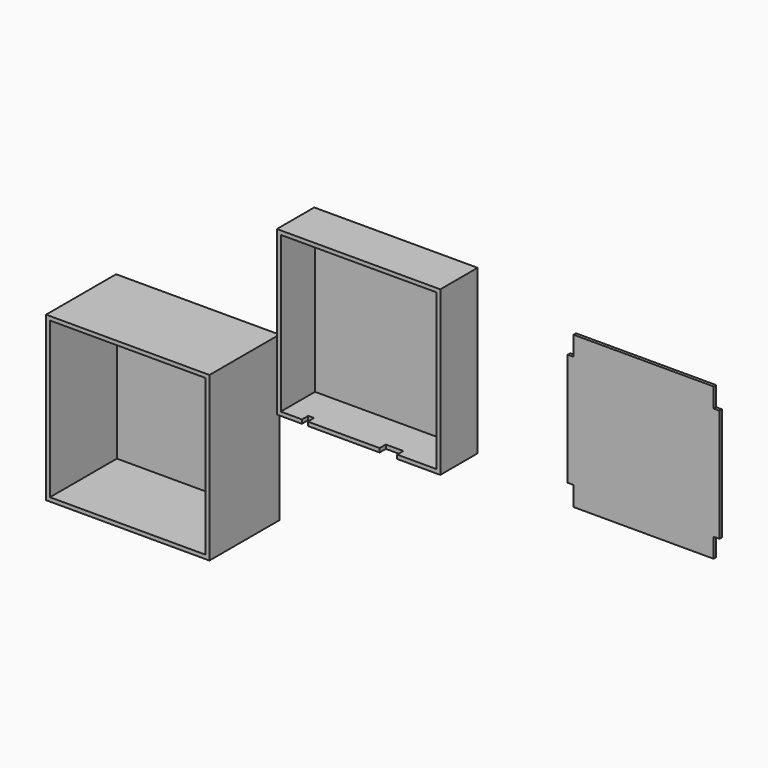
from build123d import *

# Parameters (mm, degrees)
F0_W          = 84
F0_H          = 84
F1_DEPTH      = 24
F2_W          = 80
F2_H          = 80
F3_DEPTH      = 22
F4_W          = 3
F4_H          = 4
F4_W_2        = 9
F5_DEPTH      = 2.5
F7_DEPTH      = 1.6
F8_W          = 84
F8_H          = 84
F8_W_2        = 80
F8_H_2        = 80
F9_DEPTH      = 2
F10_DEPTH     = 45
F11_TEXT_SIZE = 6.5938594684
F12_DEPTH     = 0.5


# Not quite as in the source:
# - Text() gives the source's letters only with a copy of the font that has no kerning and outlines rounded to 1/6400 em; it was checked with that copy


with BuildPart() as f1:
    # F0 (on Front) → F1 (new body)
    with BuildSketch(Plane.XZ):
        Rectangle(F0_W, F0_H)
    extrude(amount=F1_DEPTH)

    # F2 (on face) → F3 (cut)
    with BuildSketch(Plane.XZ.offset(24)):
        Rectangle(F2_W, F2_H)
    extrude(amount=-F3_DEPTH, mode=Mode.SUBTRACT)

    # F4 (on face) → F5 (cut)
    with BuildSketch(Plane(origin=(0, 0, -42), x_dir=(1, 0, 0), z_dir=(0, 0, -1))):
        with Locations((-27.5997847915, 22)):
            Rectangle(F4_W, F4_H)
        with Locations((15.3073710189, 22)):
            Rectangle(F4_W_2, F4_H)
    extrude(amount=-F5_DEPTH, mode=Mode.SUBTRACT)


with BuildPart() as f7:
    # F6 (on Front) → F7 (new body)
    with BuildSketch(Plane.XZ):
        Polygon((164.6030169576, 28.8080321075), (92.6030169576, 28.8080321075), (92.6030169576, 18.8080321075), (89.6030169576, 18.8080321075), (89.6030169576, -39.1919678925), (92.6030169576, -39.1919678925), (92.6030169576, -49.1919678925), (164.6030169576, -49.1919678925), (164.6030169576, -39.1919678925), (167.6030169576, -39.1919678925), (167.6030169576, 18.8080321075), (164.6030169576, 18.8080321075), align=None)
    extrude(amount=F7_DEPTH)


with BuildPart() as f9:
    # F8 (on Front) → F9 (new body)
    with BuildSketch(Plane.XZ):
        with Locations((-101.8717294148, -63.3563270569)):
            Rectangle(F8_W, F8_H)
        with Locations((-101.8717294148, -63.3563270569)):
            Rectangle(F8_W_2, F8_H_2, mode=Mode.SUBTRACT)
        with Locations((-101.8717294148, -63.3563270569)):
            Rectangle(F8_W_2, F8_H_2)
    extrude(amount=F9_DEPTH)

    # F8 (on Front) → F10 (join)
    with BuildSketch(Plane.XZ):
        with Locations((-101.8717294148, -63.3563270569)):
            Rectangle(F8_W, F8_H)
        with Locations((-101.8717294148, -63.3563270569)):
            Rectangle(F8_W_2, F8_H_2, mode=Mode.SUBTRACT)
    extrude(amount=F10_DEPTH)

    # F11 (on face) → F12 (cut)
    with BuildSketch(Plane(origin=(0, 0, 0), x_dir=(-1, 0, 0), z_dir=(0, 1, 0))):
        with Locations((120.8717294148, -29.1039058741)):
            Text('hubot', F11_TEXT_SIZE, font='Open Sans', font_style=FontStyle.BOLD, text_align=(TextAlign.LEFT, TextAlign.BOTTOM))
    extrude(amount=-F12_DEPTH, mode=Mode.SUBTRACT)


solid = Compound([f1.part, f7.part, f9.part])
